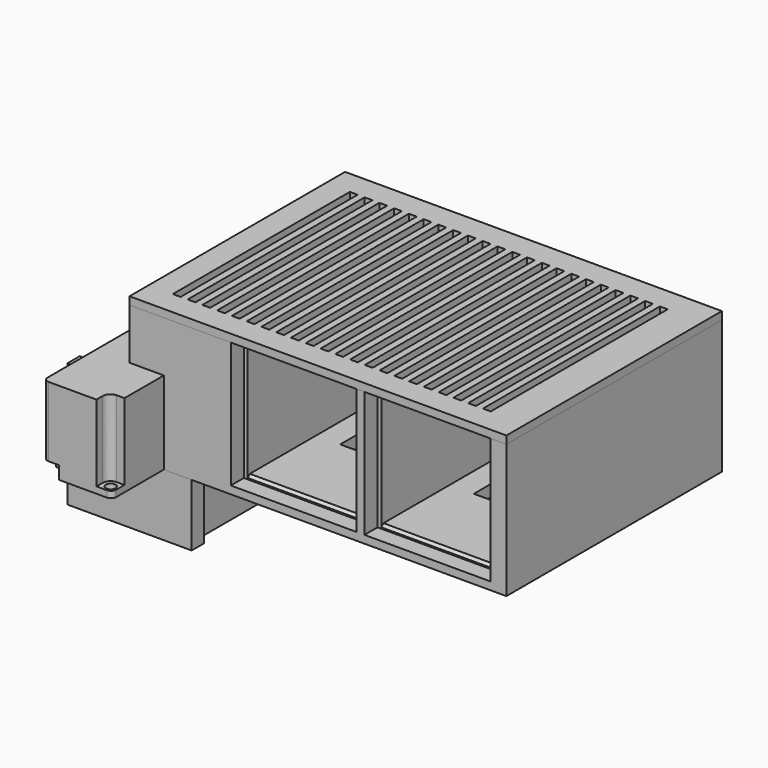
from build123d import *

# Parameters (mm, degrees)
F11_W     = 42
F11_H     = 42
F12_DEPTH = 88
F11_W_2   = 45
F11_H_2   = 45
F13_DEPTH = 80
F11_W_3   = 48
F11_H_3   = 48
F14_DEPTH = 6
F15_W     = 27
F15_H     = 35
F16_DEPTH = 45
F18_DEPTH = 32
F17_R     = 1.9
F19_DEPTH = 2.5
F20_DEPTH = 5
F21_W     = 27
F21_H     = 35
F21_W_2   = 12
F21_H_2   = 12
F21_R     = 1.25
F21_W_3   = 42.6
F21_H_3   = 8
F21_W_4   = 48.6
F21_H_4   = 3
F21_W_5   = 3
F22_DEPTH = 3
F23_DEPTH = 10
F24_DEPTH = 4.5
F25_DEPTH = 6
F26_SIZE  = 1
F27_DEPTH = 51.6
F28_W     = 3
F28_H     = 85.4
F28_W_2   = 100.2
F28_H_2   = 3.3
F29_DEPTH = 3
F30_DEPTH = 10
F31_R     = 2.5
F31_R_2   = 4.5
F32_DEPTH = 3


with BuildPart() as f12:
    # F11 (on Front) → F12 (new body)
    with BuildSketch(Plane.XZ):
        Rectangle(F11_W, F11_H)
    extrude(amount=-F12_DEPTH)

    # F11 (on Front) → F13 (join)
    with BuildSketch(Plane.XZ):
        Rectangle(F11_W_2, F11_H_2)
        Rectangle(F11_W, F11_H, mode=Mode.SUBTRACT)
    extrude(amount=-F13_DEPTH)

    # F11 (on Front) → F14 (join)
    with BuildSketch(Plane.XZ):
        Rectangle(F11_W_3, F11_H_3)
        Rectangle(F11_W_2, F11_H_2, mode=Mode.SUBTRACT)
    extrude(amount=-F14_DEPTH)

    # F15 (on face) → F16 (cut, through all)
    with BuildSketch(Plane.XY.offset(22.5)):
        with Locations((0, 56.5)):
            Rectangle(F15_W, F15_H)
    extrude(amount=-F16_DEPTH, mode=Mode.SUBTRACT)


with BuildPart() as f18:
    # F17 (on Top) → F18 (new body)
    with BuildSketch(Plane.XY):
        with BuildLine():
            Line((10.25, 19), (13.25, 19))
            Line((13.25, 19), (13.25, 23))
            ThreePointArc((13.25, 23), (12.6642135624, 24.4142135624), (11.25, 25))
            Line((11.25, 25), (7.25, 25))
            Line((7.25, 25), (7.25, 22))
            ThreePointArc((7.25, 22), (8.1286796564, 19.8786796564), (10.25, 19))
        make_face()
        with BuildLine():
            Line((-7.25, -25), (7.25, -25))
            Line((7.25, -25), (7.25, -22))
            ThreePointArc((7.25, -22), (8.1286796564, -19.8786796564), (10.25, -19))
            Line((10.25, -19), (13.25, -19))
            Line((13.25, -19), (13.25, 19))
            Line((13.25, 19), (10.25, 19))
            ThreePointArc((10.25, 19), (8.1286796564, 19.8786796564), (7.25, 22))
            Line((7.25, 22), (7.25, 25))
            Line((7.25, 25), (-7.25, 25))
            Line((-7.25, 25), (-7.25, 22))
            ThreePointArc((-7.25, 22), (-8.1286796564, 19.8786796564), (-10.25, 19))
            Line((-10.25, 19), (-13.25, 19))
            Line((-13.25, 19), (-13.25, -19))
            Line((-13.25, -19), (-10.25, -19))
            ThreePointArc((-10.25, -19), (-8.1286796564, -19.8786796564), (-7.25, -22))
            Line((-7.25, -22), (-7.25, -25))
        make_face()
        with BuildLine():
            Line((-11.25, -25), (-7.25, -25))
            Line((-7.25, -25), (-7.25, -22))
            ThreePointArc((-7.25, -22), (-8.1286796564, -19.8786796564), (-10.25, -19))
            Line((-10.25, -19), (-13.25, -19))
            Line((-13.25, -19), (-13.25, -23))
            ThreePointArc((-13.25, -23), (-12.6642135624, -24.4142135624), (-11.25, -25))
        make_face()
    extrude(amount=F18_DEPTH)

    # F17 (on Top) → F19 (join)
    with BuildSketch(Plane.XY):
        with BuildLine():
            Line((7.25, -25), (11.25, -25))
            ThreePointArc((11.25, -25), (12.6642135624, -24.4142135624), (13.25, -23))
            Line((13.25, -23), (13.25, -19))
            Line((13.25, -19), (10.25, -19))
            ThreePointArc((10.25, -19), (8.1286796564, -19.8786796564), (7.25, -22))
            Line((7.25, -22), (7.25, -25))
        make_face()
        with Locations((10.6136038969, -22.3636038969)):
            Circle(F17_R, mode=Mode.SUBTRACT)
        with BuildLine():
            Line((-13.25, 23), (-13.25, 19))
            Line((-13.25, 19), (-10.25, 19))
            ThreePointArc((-10.25, 19), (-8.1286796564, 19.8786796564), (-7.25, 22))
            Line((-7.25, 22), (-7.25, 25))
            Line((-7.25, 25), (-11.25, 25))
            ThreePointArc((-11.25, 25), (-12.6642135624, 24.4142135624), (-13.25, 23))
        make_face()
        with Locations((-10.6136038969, 22.3636038969)):
            Circle(F17_R, mode=Mode.SUBTRACT)
    extrude(amount=F19_DEPTH)

    # F17 (on Top) → F20 (cut)
    with BuildSketch(Plane.XY):
        with BuildLine():
            Line((10.25, 19), (13.25, 19))
            Line((13.25, 19), (13.25, 23))
            ThreePointArc((13.25, 23), (12.6642135624, 24.4142135624), (11.25, 25))
            Line((11.25, 25), (7.25, 25))
            Line((7.25, 25), (7.25, 22))
            ThreePointArc((7.25, 22), (8.1286796564, 19.8786796564), (10.25, 19))
        make_face()
        with BuildLine():
            Line((-11.25, -25), (-7.25, -25))
            Line((-7.25, -25), (-7.25, -22))
            ThreePointArc((-7.25, -22), (-8.1286796564, -19.8786796564), (-10.25, -19))
            Line((-10.25, -19), (-13.25, -19))
            Line((-13.25, -19), (-13.25, -23))
            ThreePointArc((-13.25, -23), (-12.6642135624, -24.4142135624), (-11.25, -25))
        make_face()
    extrude(amount=F20_DEPTH, mode=Mode.SUBTRACT)


with BuildPart() as f22:
    # F21 (on Top) → F22 (new body)
    with BuildSketch(Plane.XY):
        Polygon((40.6, 80.3), (40.6, 6.3), (86.2, 6.3), (86.2, 80.3), (84.7, 80.3), (42.1, 80.3), align=None)
        with Locations((63.4, 56.8)):
            Rectangle(F21_W, F21_H, mode=Mode.SUBTRACT)
        Polygon((92.2, 80.3), (92.2, 6.3), (137.8, 6.3), (137.8, 80.3), (136.3, 80.3), (93.7, 80.3), align=None)
        with Locations((115, 56.8)):
            Rectangle(F21_W, F21_H, mode=Mode.SUBTRACT)
        Polygon((3, 3), (37.6, 3), (37.6, 31.57279), (4.373, 31.57279), (4.373, 84.3), (37.6, 84.3), (37.6, 80.3), (40.6, 80.3), (42.1, 80.3), (42.1, 88.3), (84.7, 88.3), (84.7, 80.3), (86.2, 80.3), (92.2, 80.3), (93.7, 80.3), (93.7, 88.3), (136.3, 88.3), (136.3, 80.3), (137.8, 80.3), (142.5, 80.3), (142.5, 101), (3, 101), align=None)
        with Locations((20.9865, 20.57279)):
            Rectangle(F21_W_2, F21_H_2, mode=Mode.SUBTRACT)
        Polygon((4.373, 31.57279), (37.6, 31.57279), (37.6, 80.3), (37.6, 84.3), (4.373, 84.3), align=None)
        with Locations((31.6, 35.57279)):
            Circle(F21_R, mode=Mode.SUBTRACT)
        with Locations((10.373, 80.3)):
            Circle(F21_R, mode=Mode.SUBTRACT)
        Polygon((0, 104), (0, 0), (39.1, 0), (39.1, 3), (37.6, 3), (3, 3), (3, 101), (142.5, 101), (142.5, 80.3), (142.5, 3), (139.3, 3), (139.3, 0), (145.5, 0), (145.5, 104), align=None)
        Polygon((87.7, 6.3), (87.7, 3), (90.7, 3), (90.7, 6.3), (92.2, 6.3), (92.2, 80.3), (86.2, 80.3), (86.2, 6.3), align=None)
        Polygon((139.3, 6.3), (139.3, 3), (142.5, 3), (142.5, 80.3), (137.8, 80.3), (137.8, 6.3), align=None)
        with Locations((63.4, 84.3)):
            Rectangle(F21_W_3, F21_H_3)
        with Locations((115, 84.3)):
            Rectangle(F21_W_3, F21_H_3)
        Polygon((37.6, 3), (39.1, 3), (39.1, 6.3), (40.6, 6.3), (40.6, 80.3), (37.6, 80.3), (37.6, 31.57279), align=None)
        Polygon((39.1, 6.3), (39.1, 3), (87.7, 3), (87.7, 6.3), (86.2, 6.3), (40.6, 6.3), align=None)
        Polygon((90.7, 6.3), (90.7, 3), (139.3, 3), (139.3, 6.3), (137.8, 6.3), (92.2, 6.3), align=None)
        with Locations((63.4, 1.5)):
            Rectangle(F21_W_4, F21_H_4)
        with Locations((115, 1.5)):
            Rectangle(F21_W_4, F21_H_4)
        with Locations((89.2, 1.5)):
            Rectangle(F21_W_5, F21_H_4)
        with Locations((10.373, 80.3)):
            Circle(F21_R)
        with Locations((31.6, 35.57279)):
            Circle(F21_R)
    extrude(amount=F22_DEPTH)

    # F21 (on Top) → F23 (join)
    with BuildSketch(Plane.XY):
        Polygon((4.373, 31.57279), (37.6, 31.57279), (37.6, 80.3), (37.6, 84.3), (4.373, 84.3), align=None)
        with Locations((31.6, 35.57279)):
            Circle(F21_R, mode=Mode.SUBTRACT)
        with Locations((10.373, 80.3)):
            Circle(F21_R, mode=Mode.SUBTRACT)
    extrude(amount=F23_DEPTH)

    # F21 (on Top) → F24 (join)
    with BuildSketch(Plane.XY):
        Polygon((40.6, 80.3), (40.6, 6.3), (86.2, 6.3), (86.2, 80.3), (84.7, 80.3), (42.1, 80.3), align=None)
        with Locations((63.4, 56.8)):
            Rectangle(F21_W, F21_H, mode=Mode.SUBTRACT)
        Polygon((92.2, 80.3), (92.2, 6.3), (137.8, 6.3), (137.8, 80.3), (136.3, 80.3), (93.7, 80.3), align=None)
        with Locations((115, 56.8)):
            Rectangle(F21_W, F21_H, mode=Mode.SUBTRACT)
    extrude(amount=F24_DEPTH)

    # F21 (on Top) → F25 (join)
    with BuildSketch(Plane.XY):
        with Locations((63.4, 84.3)):
            Rectangle(F21_W_3, F21_H_3)
        with Locations((115, 84.3)):
            Rectangle(F21_W_3, F21_H_3)
    extrude(amount=F25_DEPTH)

    # F26
    f26_edges = [f22.edges().sort_by_distance(p)[0] for p in [
        (63.4, 80.3, 6),
        (115, 80.3, 6),
        (63.4, 6.3, 4.5),
        (115, 6.3, 4.5),
    ]]
    chamfer(f26_edges, length=F26_SIZE)

    # F21 (on Top) → F27 (join)
    with BuildSketch(Plane.XY):
        Polygon((0, 104), (0, 0), (39.1, 0), (39.1, 3), (37.6, 3), (3, 3), (3, 101), (142.5, 101), (142.5, 80.3), (142.5, 3), (139.3, 3), (139.3, 0), (145.5, 0), (145.5, 104), align=None)
        with Locations((89.2, 1.5)):
            Rectangle(F21_W_5, F21_H_4)
        Polygon((139.3, 6.3), (139.3, 3), (142.5, 3), (142.5, 80.3), (137.8, 80.3), (137.8, 6.3), align=None)
        Polygon((87.7, 6.3), (87.7, 3), (90.7, 3), (90.7, 6.3), (92.2, 6.3), (92.2, 80.3), (86.2, 80.3), (86.2, 6.3), align=None)
        Polygon((37.6, 3), (39.1, 3), (39.1, 6.3), (40.6, 6.3), (40.6, 80.3), (37.6, 80.3), (37.6, 31.57279), align=None)
    extrude(amount=F27_DEPTH)

    # F31 (on face) → F32 (cut, through all)
    with BuildSketch(Plane(origin=(0, 0, 0), x_dir=(0, -1, 0), z_dir=(-1, 0, 0))):
        with Locations((-95, 36)):
            Circle(F31_R)
        with Locations((-95, 24)):
            Circle(F31_R_2)
        with Locations((-95, 9)):
            Circle(F31_R_2)
    extrude(amount=-F32_DEPTH, mode=Mode.SUBTRACT)


with BuildPart() as f29:
    # F28 (on face) → F29 (new body)
    with BuildSketch(Plane.XY.offset(51.6)):
        Polygon((139.3, 0), (145.5, 0), (145.5, 104), (0, 104), (0, 0), (39.1, 0), (39.1, 3.3), (37.6, 3.3), (37.6, 3), (3, 3), (3, 101), (142.5, 101), (142.5, 80.3), (142.2, 80.3), (142.2, 3.3), (139.3, 3.3), align=None)
        Polygon((3.3, 100.7), (3.3, 88.6), (6.3, 88.6), (6.3, 97.7), (15.4, 97.7), (15.4, 100.7), align=None)
        Polygon((139.2, 88.6), (142.2, 88.6), (142.2, 100.7), (130.1, 100.7), (130.1, 97.7), (139.2, 97.7), align=None)
        Polygon((3.3, 3.3), (15.4, 3.3), (15.4, 6.3), (6.3, 6.3), (6.3, 15.4), (3.3, 15.4), align=None)
        Polygon((39.1, 3.3), (139.3, 3.3), (139.3, 6.3), (137.8, 6.3), (137.8, 80.3), (142.2, 80.3), (142.2, 88.6), (139.2, 88.6), (139.2, 97.7), (130.1, 97.7), (130.1, 100.7), (15.4, 100.7), (15.4, 97.7), (6.3, 97.7), (6.3, 88.6), (3.3, 88.6), (3.3, 15.4), (6.3, 15.4), (6.3, 6.3), (15.4, 6.3), (15.4, 3.3), (37.6, 3.3), (37.6, 80.3), (37.8, 80.3), (37.8, 94.7), (40.8, 94.7), (40.8, 9.3), (40.6, 9.3), (40.6, 6.3), (39.1, 6.3), align=None)
        with Locations((10.8, 52)):
            Rectangle(F28_W, F28_H, mode=Mode.SUBTRACT)
        with Locations((16.5, 52)):
            Rectangle(F28_W, F28_H, mode=Mode.SUBTRACT)
        with Locations((22.2, 52)):
            Rectangle(F28_W, F28_H, mode=Mode.SUBTRACT)
        with Locations((27.9, 52)):
            Rectangle(F28_W, F28_H, mode=Mode.SUBTRACT)
        with Locations((33.6, 52)):
            Rectangle(F28_W, F28_H, mode=Mode.SUBTRACT)
        with Locations((45, 52)):
            Rectangle(F28_W, F28_H, mode=Mode.SUBTRACT)
        with Locations((50.7, 52)):
            Rectangle(F28_W, F28_H, mode=Mode.SUBTRACT)
        with Locations((56.4, 52)):
            Rectangle(F28_W, F28_H, mode=Mode.SUBTRACT)
        with Locations((62.1, 52)):
            Rectangle(F28_W, F28_H, mode=Mode.SUBTRACT)
        with Locations((67.8, 52)):
            Rectangle(F28_W, F28_H, mode=Mode.SUBTRACT)
        with Locations((73.5, 52)):
            Rectangle(F28_W, F28_H, mode=Mode.SUBTRACT)
        with Locations((79.2, 52)):
            Rectangle(F28_W, F28_H, mode=Mode.SUBTRACT)
        with Locations((84.9, 52)):
            Rectangle(F28_W, F28_H, mode=Mode.SUBTRACT)
        with Locations((90.6, 52)):
            Rectangle(F28_W, F28_H, mode=Mode.SUBTRACT)
        with Locations((96.3, 52)):
            Rectangle(F28_W, F28_H, mode=Mode.SUBTRACT)
        with Locations((102, 52)):
            Rectangle(F28_W, F28_H, mode=Mode.SUBTRACT)
        with Locations((107.7, 52)):
            Rectangle(F28_W, F28_H, mode=Mode.SUBTRACT)
        with Locations((113.4, 52)):
            Rectangle(F28_W, F28_H, mode=Mode.SUBTRACT)
        with Locations((119.1, 52)):
            Rectangle(F28_W, F28_H, mode=Mode.SUBTRACT)
        with Locations((124.8, 52)):
            Rectangle(F28_W, F28_H, mode=Mode.SUBTRACT)
        with Locations((130.5, 52)):
            Rectangle(F28_W, F28_H, mode=Mode.SUBTRACT)
        Polygon((37.6, 3.3), (39.1, 3.3), (39.1, 6.3), (40.6, 6.3), (40.6, 9.3), (37.8, 9.3), (37.8, 80.3), (37.6, 80.3), align=None)
        Polygon((139.3, 6.3), (139.3, 3.3), (142.2, 3.3), (142.2, 80.3), (137.8, 80.3), (137.8, 6.3), align=None)
        with Locations((89.2, 1.65)):
            Rectangle(F28_W_2, F28_H_2)
        Polygon((37.6, 3), (37.6, 3.3), (15.4, 3.3), (3.3, 3.3), (3.3, 15.4), (3.3, 88.6), (3.3, 100.7), (15.4, 100.7), (130.1, 100.7), (142.2, 100.7), (142.2, 88.6), (142.2, 80.3), (142.5, 80.3), (142.5, 101), (3, 101), (3, 3), align=None)
    extrude(amount=F29_DEPTH)

    # F28 (on face) → F30 (join)
    with BuildSketch(Plane.XY.offset(51.6)):
        Polygon((3.3, 100.7), (3.3, 88.6), (6.3, 88.6), (6.3, 97.7), (15.4, 97.7), (15.4, 100.7), align=None)
        Polygon((3.3, 3.3), (15.4, 3.3), (15.4, 6.3), (6.3, 6.3), (6.3, 15.4), (3.3, 15.4), align=None)
        Polygon((139.2, 88.6), (142.2, 88.6), (142.2, 100.7), (130.1, 100.7), (130.1, 97.7), (139.2, 97.7), align=None)
    extrude(amount=-F30_DEPTH)


solid = Compound([f12.part, f18.part, f22.part, f29.part])
